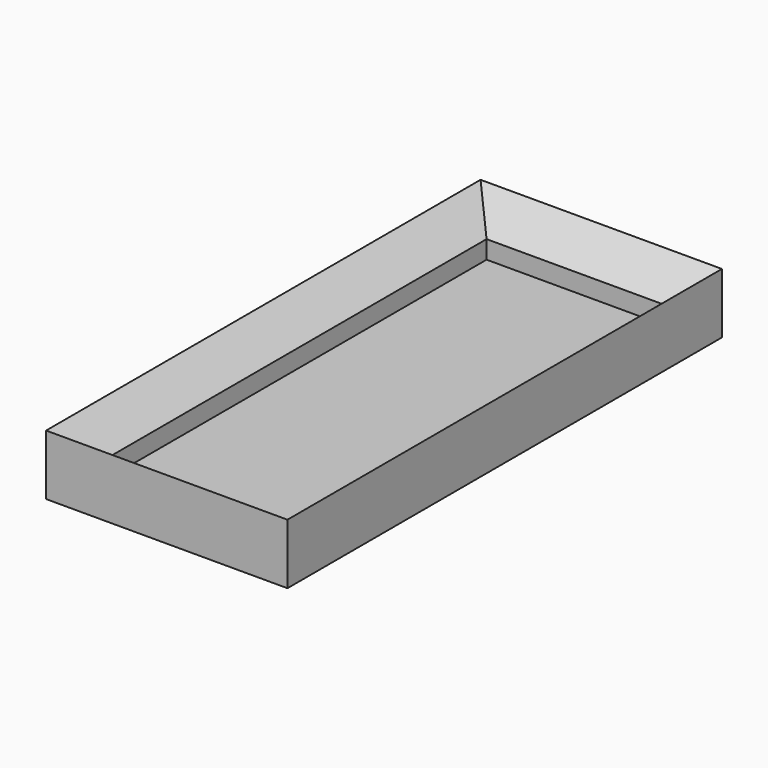
from build123d import *

# Parameters (mm, degrees)
F0_W     = 40
F0_H     = 90
F0_W_2   = 30
F0_H_2   = 80
F1_DEPTH = 10
F2_DEPTH = 2
F3_SIZE  = 4.99999


# Not quite as in the source:
# - a fillet or chamfer is up to 0.001 mm smaller than in the source, because OpenCascade refuses the exact size


with BuildPart() as f1:
    # F0 (on Top) → F1 (new body)
    with BuildSketch(Plane.XY):
        with Locations((1.4284082502, 37.2216339977)):
            Rectangle(F0_W, F0_H)
        with Locations((1.4284082502, 37.2216339977)):
            Rectangle(F0_W_2, F0_H_2, mode=Mode.SUBTRACT)
    extrude(amount=F1_DEPTH)

    # F0 (on Top) → F2 (join)
    with BuildSketch(Plane.XY):
        with Locations((1.4284082502, 37.2216339977)):
            Rectangle(F0_W_2, F0_H_2)
    extrude(amount=F2_DEPTH)

    # F3 (size 5 in the source; OpenCascade refuses exactly that, so slightly less here)
    f3_edges = [f1.edges().sort_by_distance(p)[0] for p in [
        (16.428408, 37.221634, 10),
        (1.428408, 77.221634, 10),
        (-13.571592, 37.221634, 10),
        (1.428408, -2.778366, 10),
    ]]
    chamfer(f3_edges, length=F3_SIZE)


solid = f1.part
